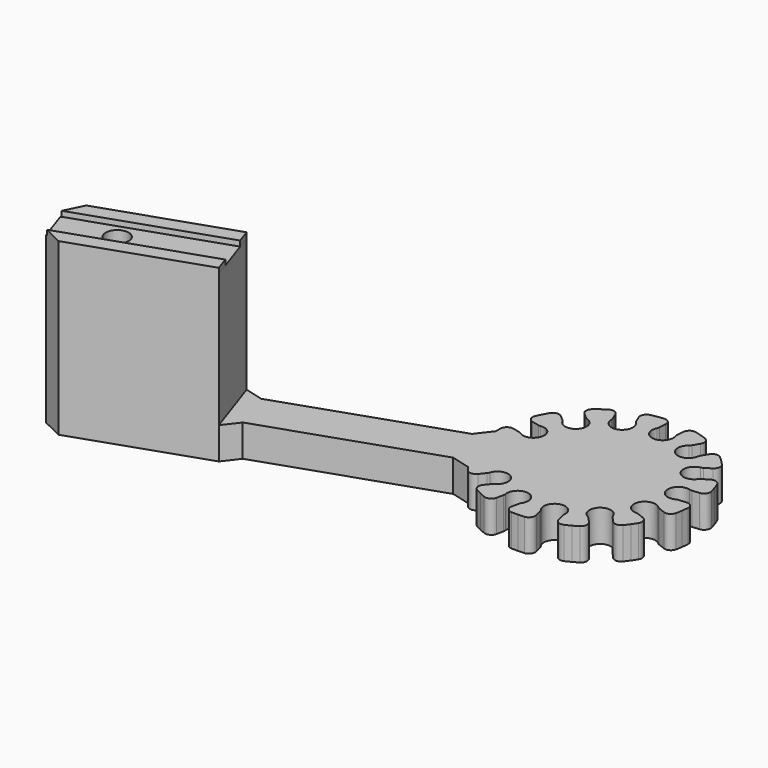
from build123d import *

# Parameters (mm, degrees)
F0_R         = 2.15
F1_DEPTH     = 6
F2_R         = 2.15
F3_DEPTH     = 25
F5_DEPTH     = 1
F7_R         = 4
F8_DEPTH     = 25
F10_DEPTH    = 6
F11_T1_DEPTH = 47.4300979278


# Not quite as in the source:
# - a fillet or chamfer that OpenCascade refuses, or shapes differently, is made with other operations: its cross-section is extruded or revolved along the edge and cut away or added


with BuildPart() as f1:
    # F0 (on Top) → F1 (new body)
    with BuildSketch(Plane.XY):
        with BuildLine():
            ThreePointArc((-18.5969470694, 1.1730885182), (-18.6246664736, 0.5868353432), (-18.6339093315, 0))
            Line((-18.6339093315, 0), (-81.8843098804, -21.5119105478))
            Line((-81.8843098804, -21.5119105478), (-78.0203863891, -32.8728125918))
            Line((-78.0203863891, -32.8728125918), (-14.7699858402, -11.360902044))
            ThreePointArc((-14.7699858402, -11.360902044), (-14.4048721322, -11.8204160598), (-14.0254681126, -12.2682036662))
            ThreePointArc((-14.0254681126, -12.2682036662), (-13.0994365935, -12.6779301983), (-12.189647328, -12.2333026039))
            Line((-12.189647328, -12.2333026039), (-11.3302968808, -11.1720260314))
            ThreePointArc((-11.3302968808, -11.1720260314), (-11.2052452091, -10.9837708237), (-11.1177092299, -10.7754072085))
            ThreePointArc((-11.1177092299, -10.7754072085), (-7.9504729238, -9.8186376491), (-8.2276252662, -13.1156029792))
            ThreePointArc((-8.2276252662, -13.1156029792), (-8.4132279023, -13.2445588061), (-8.5713595843, -13.4060280444))
            Line((-8.5713595843, -13.4060280444), (-9.4307100315, -14.467304617))
            ThreePointArc((-9.4307100315, -14.467304617), (-9.6764048229, -15.4496712873), (-9.0830482328, -16.2702431382))
            ThreePointArc((-9.0830482328, -16.2702431382), (-8.5661461233, -16.5482240004), (-8.0407459935, -16.809788245))
            ThreePointArc((-8.0407459935, -16.809788245), (-7.5073690649, -17.054676388), (-6.9665444726, -17.2826454886))
            ThreePointArc((-6.9665444726, -17.2826454886), (-5.9553088883, -17.2296096656), (-5.344694665, -16.4217975117))
            Line((-5.344694665, -16.4217975117), (-5.0577736002, -15.0867067069))
            ThreePointArc((-5.0577736002, -15.0867067069), (-5.0313061862, -14.8622575595), (-5.0473923975, -14.6368264666))
            ThreePointArc((-5.0473923975, -14.6368264666), (-2.6545144237, -12.3518912791), (-1.4116534913, -15.4181741282))
            ThreePointArc((-1.4116534913, -15.4181741282), (-1.518935585, -15.6170924436), (-1.587017804, -15.8325982562))
            Line((-1.587017804, -15.8325982562), (-1.8739388688, -17.167689061))
            ThreePointArc((-1.8739388688, -17.167689061), (-1.649119192, -18.1550422493), (-0.7489575534, -18.618851725))
            ThreePointArc((-0.7489575534, -18.618851725), (-0.1622249168, -18.6332031613), (0.4246686545, -18.6290695825))
            ThreePointArc((0.4246686545, -18.6290695825), (1.0111409345, -18.6064550892), (1.596610115, -18.565382116))
            ThreePointArc((1.596610115, -18.565382116), (2.4747016485, -18.0610355443), (2.6542957209, -17.0644633319))
            Line((2.6542957209, -17.0644633319), (2.3068348031, -15.7438339118))
            ThreePointArc((2.3068348031, -15.7438339118), (2.2290030596, -15.5316543569), (2.1127680264, -15.3378313426))
            ThreePointArc((2.1127680264, -15.3378313426), (3.2146124186, -12.2180985425), (5.7091254771, -14.3916206633))
            ThreePointArc((5.7091254771, -14.3916206633), (5.7033285013, -14.6175506057), (5.7399962013, -14.8405605238))
            Line((5.7399962013, -14.8405605238), (6.0874571192, -16.1611899438))
            ThreePointArc((6.0874571192, -16.1611899438), (6.7342477263, -16.9403382712), (7.7468496176, -16.9472386534))
            ThreePointArc((7.7468496176, -16.9472386534), (8.2767242352, -16.6948618715), (8.7983879526, -16.4259230002))
            ThreePointArc((8.7983879526, -16.4259230002), (9.3113232547, -16.1406888397), (9.8150212856, -15.8394423556))
            ThreePointArc((9.8150212856, -15.8394423556), (10.3703693959, -14.9926846087), (10.0801649873, -14.0225343076))
            Line((10.0801649873, -14.0225343076), (9.1733465796, -13.0015193567))
            ThreePointArc((9.1733465796, -13.0015193567), (9.0080212726, -12.8474236505), (8.8167351306, -12.727059388))
            ThreePointArc((8.8167351306, -12.727059388), (8.3896333805, -9.4461482487), (11.5971780544, -10.2575981694))
            ThreePointArc((11.5971780544, -10.2575981694), (11.6941178917, -10.4617564701), (11.8276181438, -10.6441177228))
            Line((11.8276181438, -10.6441177228), (12.7344365515, -11.6651326736))
            ThreePointArc((12.7344365515, -11.6651326736), (13.6635416995, -12.0678407931), (14.5699407115, -11.6163421368))
            ThreePointArc((14.5699407115, -11.6163421368), (14.9285456674, -11.1517308626), (15.2723408028, -10.6760565461))
            ThreePointArc((15.2723408028, -10.6760565461), (15.6009850569, -10.1897910787), (15.914152399, -9.6934168587))
            ThreePointArc((15.914152399, -9.6934168587), (16.026845153, -8.6870816517), (15.3295038103, -7.9528301572))
            Line((15.3295038103, -7.9528301572), (14.0591300522, -7.451889373))
            ThreePointArc((14.0591300522, -7.451889373), (13.8420085699, -7.3891501848), (13.6169742256, -7.368233979))
            ThreePointArc((13.6169742256, -7.368233979), (11.7531470422, -4.6345657403), (14.9811435333, -3.9087334858))
            ThreePointArc((14.9811435333, -3.9087334858), (15.15988873, -4.0470378548), (15.3613958788, -4.1493746165))
            Line((15.3613958788, -4.1493746165), (16.6317696368, -4.6503154007))
            ThreePointArc((16.6317696368, -4.6503154007), (17.6425749863, -4.5896297274), (18.2470595362, -3.7772205728))
            ThreePointArc((18.2470595362, -3.7772205728), (18.3569640934, -3.2006946507), (18.4486576776, -2.6209934888))
            ThreePointArc((18.4486576776, -2.6209934888), (18.5220493245, -2.0386921779), (18.577066226, -1.4543683883))
            ThreePointArc((18.577066226, -1.4543683883), (18.2227707671, -0.5057457377), (17.2688639009, -0.1659341781))
            Line((17.2688639009, -0.1659341781), (15.9092365685, -0.2932317491))
            ThreePointArc((15.9092365685, -0.2932317491), (15.6872002385, -0.3353958565), (15.4770075811, -0.4184439786))
            ThreePointArc((15.4770075811, -0.4184439786), (12.5788964533, 1.1777219588), (15.1303489642, 3.2841131601))
            ThreePointArc((15.1303489642, 3.2841131601), (15.3523044812, 3.2415256934), (15.5783086788, 3.2413101917))
            Line((15.5783086788, 3.2413101917), (16.9379360112, 3.3686077628))
            ThreePointArc((16.9379360112, 3.3686077628), (17.8121863433, 3.8795838506), (17.9842348547, 4.8774864086))
            ThreePointArc((17.9842348547, 4.8774864086), (17.8217081898, 5.4414422878), (17.641501551, 6))
            ThreePointArc((17.641501551, 6), (17.4437937118, 6.5526054296), (17.2287808075, 7.098710366))
            ThreePointArc((17.2287808075, 7.098710366), (16.4839973571, 7.7847918607), (15.4794945459, 7.6567906581))
            Line((15.4794945459, 7.6567906581), (14.324187235, 6.9287410913))
            ThreePointArc((14.324187235, 6.9287410913), (14.145178609, 6.7907778511), (13.9952128796, 6.6216973264))
            ThreePointArc((13.9952128796, 6.6216973264), (10.6885840629, 6.7357134534), (12.0125775964, 9.7678471793))
            ThreePointArc((12.0125775964, 9.7678471793), (12.2298183312, 9.8301721903), (12.4315202756, 9.9321244802))
            Line((12.4315202756, 9.9321244802), (13.5868275865, 10.660174047))
            ThreePointArc((13.5868275865, 10.660174047), (14.1357529292, 11.5111095168), (13.8382163253, 12.4790362572))
            ThreePointArc((13.8382163253, 12.4790362572), (13.438351538, 12.908651553), (13.025155273, 13.3254608584))
            ThreePointArc((13.025155273, 13.3254608584), (12.5990374405, 13.729050679), (12.1604207694, 14.1190206348))
            ThreePointArc((12.1604207694, 14.1190206348), (11.1859645378, 14.394420813), (10.3477601432, 13.8262451373))
            Line((10.3477601432, 13.8262451373), (9.6462292403, 12.6546455698))
            ThreePointArc((9.6462292403, 12.6546455698), (9.5489002377, 12.4506725101), (9.4915423523, 12.2320678057))
            ThreePointArc((9.4915423523, 12.2320678057), (6.4903701015, 10.83931552), (6.3010251868, 14.1424870735))
            ThreePointArc((6.3010251868, 14.1424870735), (6.4666440625, 14.2962672146), (6.6004918453, 14.4783735431))
            Line((6.6004918453, 14.4783735431), (7.3020227482, 15.6499731106))
            ThreePointArc((7.3020227482, 15.6499731106), (7.4070979859, 16.6571321844), (6.7042209966, 17.3860863279))
            ThreePointArc((6.7042209966, 17.3860863279), (6.1533577335, 17.5885976012), (5.5963900496, 17.7736601573))
            ThreePointArc((5.5963900496, 17.7736601573), (5.0338704832, 17.9410904053), (4.4663570802, 18.0907222467))
            ThreePointArc((4.4663570802, 18.0907222467), (3.4726347083, 17.8959761222), (2.9817155877, 17.0103076613))
            Line((2.9817155877, 17.0103076613), (2.8854371221, 15.648132338))
            ThreePointArc((2.8854371221, 15.648132338), (2.890803226, 15.4221917512), (2.93843802, 15.201264455))
            ThreePointArc((2.93843802, 15.201264455), (0.890741765, 12.6024697621), (-0.7710578453, 15.463451388))
            ThreePointArc((-0.7710578453, 15.463451388), (-0.6928216048, 15.6754821274), (-0.6557286787, 15.8984217126))
            Line((-0.6557286787, 15.8984217126), (-0.5594502131, 17.260597036))
            ThreePointArc((-0.5594502131, 17.260597036), (-0.9209131469, 18.2065118064), (-1.8773638425, 18.5390960399))
            ThreePointArc((-1.8773638425, 18.5390960399), (-2.4602820261, 18.4707766303), (-3.0407594941, 18.3841333403))
            ThreePointArc((-3.0407594941, 18.3841333403), (-3.6182203854, 18.2792521241), (-4.1920918317, 18.1562370289))
            ThreePointArc((-4.1920918317, 18.1562370289), (-4.9905137175, 17.5333945948), (-5.0281472742, 16.5214687473))
            Line((-5.0281472742, 16.5214687473), (-4.4983846536, 15.2628414314))
            ThreePointArc((-4.4983846536, 15.2628414314), (-4.3914821036, 15.0637188847), (-4.2491400352, 14.8881720835))
            ThreePointArc((-4.2491400352, 14.8881720835), (-4.9012174084, 11.6444722041), (-7.6766524443, 13.4455147271))
            ThreePointArc((-7.6766524443, 13.4455147271), (-7.7026917728, 13.6700139413), (-7.7703628861, 13.8856491987))
            Line((-7.7703628861, 13.8856491987), (-8.3001255068, 15.1442765146))
            ThreePointArc((-8.3001255068, 15.1442765146), (-9.0500787744, 15.8247030733), (-10.0535843288, 15.6891051089))
            ThreePointArc((-10.0535843288, 15.6891051089), (-10.5426925115, 15.3647066871), (-11.0213418468, 15.0250657526))
            ThreePointArc((-11.0213418468, 15.0250657526), (-11.4890574918, 14.6705192452), (-11.9453754506, 14.3014188918))
            ThreePointArc((-11.9453754506, 14.3014188918), (-12.3760999161, 13.3849655976), (-11.9523219921, 12.4652795225))
            Line((-11.9523219921, 12.4652795225), (-10.9109057454, 11.5819656737))
            ThreePointArc((-10.9109057454, 11.5819656737), (-10.725549373, 11.4526561265), (-10.5192348293, 11.3603942552))
            ThreePointArc((-10.5192348293, 11.3603942552), (-9.6348954016, 8.1721756954), (-12.9246880877, 8.5243942227))
            ThreePointArc((-12.9246880877, 8.5243942227), (-13.0493805185, 8.7128875688), (-13.207203982, 8.8746580797))
            Line((-13.207203982, 8.8746580797), (-14.2486202287, 9.7579719285))
            ThreePointArc((-14.2486202287, 9.7579719285), (-15.225132342, 10.0259911406), (-16.0590137233, 9.4514895762))
            ThreePointArc((-16.0590137233, 9.4514895762), (-16.3487026368, 8.9410569324), (-16.6221728673, 8.4217543389))
            ThreePointArc((-16.6221728673, 8.4217543389), (-16.8791531193, 7.8940969685), (-17.1193884565, 7.3586082821))
            ThreePointArc((-17.1193884565, 7.3586082821), (-17.0894125683, 6.3464266523), (-16.295726185, 5.7175609031))
            Line((-16.295726185, 5.7175609031), (-14.9675211005, 5.4002875069))
            ThreePointArc((-14.9675211005, 5.4002875069), (-14.7437334438, 5.3687117488), (-14.5179942954, 5.3796561849))
            ThreePointArc((-14.5179942954, 5.3796561849), (-12.2881864976, 2.9353258076), (-15.3819978718, 1.7626685733))
            ThreePointArc((-15.3819978718, 1.7626685733), (-15.5784195529, 1.8744561711), (-15.792317792, 1.9474321063))
            Line((-15.792317792, 1.9474321063), (-17.1205228765, 2.2647055024))
            ThreePointArc((-17.1205228765, 2.2647055024), (-18.1127432844, 2.0624460954), (-18.5969470694, 1.1730885182))
        make_face()
        with Locations((-70.4849297647, -23.972425327)):
            Circle(F0_R, mode=Mode.SUBTRACT)
    extrude(amount=F1_DEPTH)

    # F2 (on face) → F3 (join)
    with BuildSketch(Plane.XY.offset(6)):
        Polygon((-55.3755384443, -12.4960890681), (-81.8843098804, -21.5119105478), (-78.0203863891, -32.8728125918), (-51.5116149531, -23.8569911122), align=None)
        with Locations((-70.4849297647, -23.972425327)):
            Circle(F2_R, mode=Mode.SUBTRACT)
    extrude(amount=F3_DEPTH)

    # F4 (on face) → F5 (join)
    with BuildSketch(Plane.XY.offset(31)):
        Polygon((-54.4739562964, -15.1469662117), (-55.3755384443, -12.4960890681), (-81.8843098804, -21.5119105478), (-80.9827277324, -24.1627876914), align=None)
        Polygon((-78.0203863891, -32.8728125918), (-51.5116149531, -23.8569911122), (-52.413197101, -21.2061139686), (-78.9219685371, -30.2219354482), align=None)
    extrude(amount=F5_DEPTH)

    # F7 (on face) → F8 (cut, through all)
    with BuildSketch(Plane(origin=(0, 0, 0), x_dir=(1, 0, 0), z_dir=(0, 0, -1))):
        with Locations((-70.4849297647, 23.972425327)):
            Circle(F7_R)
    extrude(amount=-F8_DEPTH, mode=Mode.SUBTRACT)

    # F9 (on face) → F10 (cut, through all)
    with BuildSketch(Plane.XY.offset(6)):
        Polygon((-20.8301475939, -2.8594645468), (-18.6339093315, 0), (-55.3755384443, -12.4960890681), (-51.8913256848, -13.4235918693), align=None)
        Polygon((-51.5116149531, -23.8569911122), (-14.7699858402, -11.360902044), (-18.2541985998, -10.4333992428), (-49.3153766906, -20.9975265653), align=None)
    extrude(amount=-F10_DEPTH, mode=Mode.SUBTRACT)

    # F11: chamfer of 3 on 2 edges, made by hand

    # F11_s2 → F11_t1 (cut)
    with BuildSketch(Plane.XY.offset(-7.7150489639)):
        Polygon((-75.1801608781, -31.906831719), (-78.9863672619, -30.0325870808), (-78.0203863891, -32.8728125918), align=None)
        Polygon((-80.9183290076, -24.3521360588), (-79.0440843694, -20.5459296749), (-81.8843098804, -21.5119105478), align=None)
    extrude(amount=F11_T1_DEPTH, mode=Mode.SUBTRACT)


solid = f1.part
